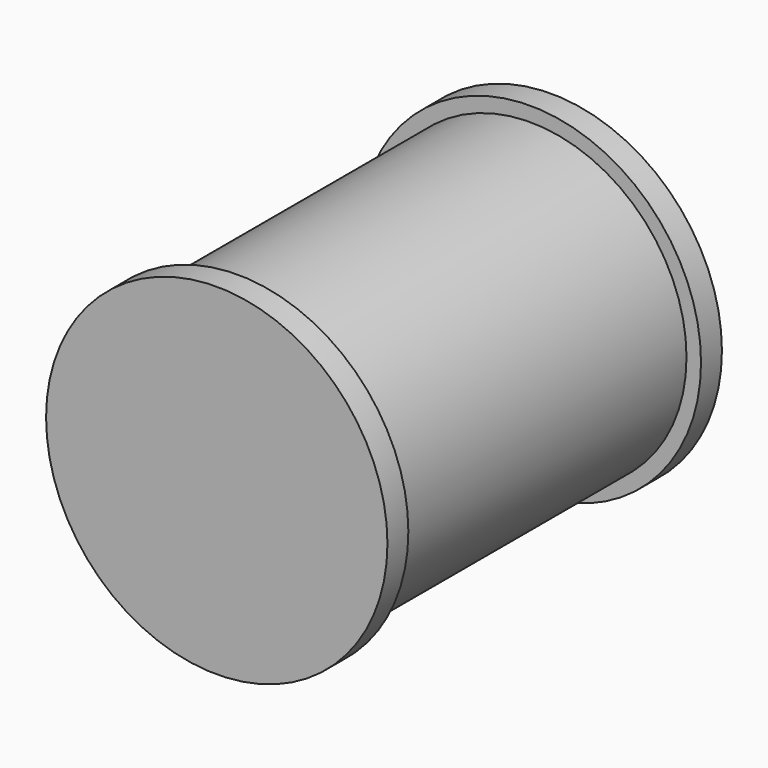
from build123d import *

# Parameters (mm, degrees)
F0_R          = 1.5180836213
F1_DEPTH      = 1.778
F1_DEPTH_BACK = 1.778
F2_R          = 1.6591021796
F3_DEPTH      = 0.254


# Not quite as in the source:
# - a pattern or mirror of a feature is missing from the dataset's text; its kind, count and spacing are read off the source's solid


with BuildPart() as f1:
    # F0 (on Front) → F1 (new body, two sides)
    with BuildSketch(Plane.XZ) as f1_sk:
        Circle(F0_R)
    extrude(amount=F1_DEPTH)
    extrude(f1_sk.sketch, amount=-F1_DEPTH_BACK)

    # F2 (on face) → F3 (join)
    with BuildSketch(Plane.XZ.offset(1.778)):
        Circle(F2_R)
    f3 = extrude(amount=F3_DEPTH)

    # F3_copies: F3 across plane
    add(f3.mirror(Plane.ZX))


solid = f1.part
